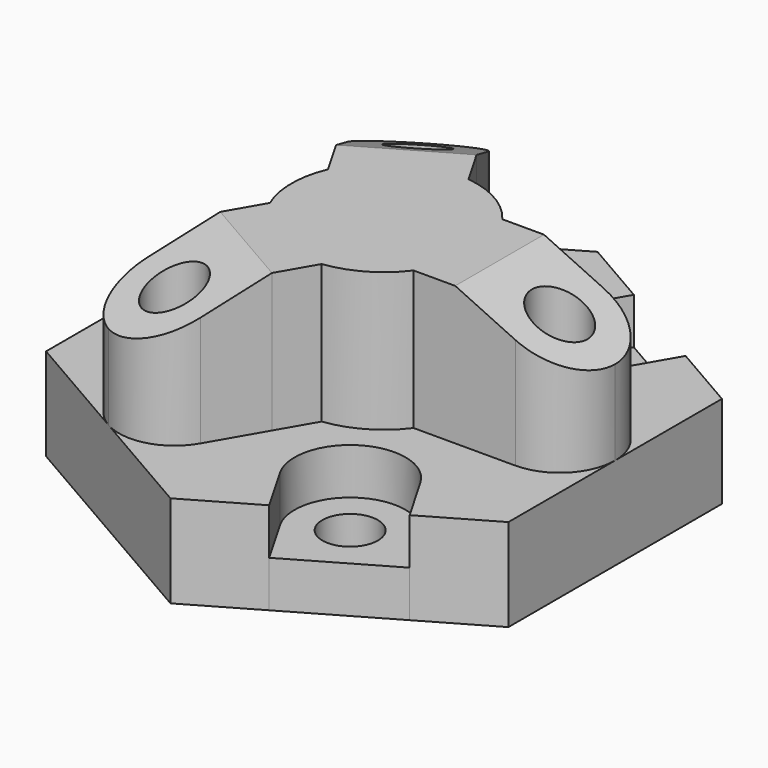
from build123d import *

# Parameters (mm, degrees)
F1_R            = 6
F2_DEPTH        = 20
F3_DEPTH        = 30
F3_DEPTH_BACK   = 20
F4_DEPTH        = 10
F6_DEPTH        = 12.5
F6_COPIES_COUNT = 3


# Not quite as in the source:
# - a pattern or mirror of a feature is missing from the dataset's text; its kind, count and spacing are read off the source's solid


with BuildPart() as f2:
    # F1 (on offset) → F2 (new body, through all)
    with BuildSketch(Plane.XY.offset(20)):
        with BuildLine():
            ThreePointArc((-29.3923048454, 26.9089653438), (-30.5911098969, 36.0147939544), (-24.9999998757, 43.301270261))
            Line((-24.9999998757, 43.301270261), (-50, 28.8675134595))
            Line((-50, 28.8675134595), (-50, 12))
            Line((-50, 12), (-38, 12))
            ThreePointArc((-38, 12), (-26, 0), (-38, -12))
            Line((-38, -12), (-50, -12))
            Line((-50, -12), (-50, -28.8675134595))
            Line((-50, -28.8675134595), (-24.9999998757, -43.301270261))
            ThreePointArc((-24.9999998757, -43.301270261), (-30.5911098969, -36.0147939544), (-29.3923048454, -26.9089653438))
            Line((-29.3923048454, -26.9089653438), (-22.8923048454, -15.6506350946))
            Line((-22.8923048454, -15.6506350946), (-18.3923048454, -7.8564064606))
            ThreePointArc((-18.3923048454, -7.8564064606), (-20, 0), (-18.3923048454, 7.8564064606))
            Line((-18.3923048454, 7.8564064606), (-22.8923048454, 15.6506350946))
            Line((-22.8923048454, 15.6506350946), (-29.3923048454, 26.9089653438))
        make_face()
        with BuildLine():
            Line((-38, 12), (-50, 12))
            Line((-50, 12), (-50, -12))
            Line((-50, -12), (-38, -12))
            ThreePointArc((-38, -12), (-26, 0), (-38, 12))
        make_face()
        with Locations((-38, 0)):
            Circle(F1_R, mode=Mode.SUBTRACT)
    extrude(amount=-F2_DEPTH)



with BuildPart() as f2b:
    # F1 (on offset) → F2, piece 2 (new body, through all)
    with BuildSketch(Plane.XY.offset(20)):
        with BuildLine():
            Line((50, -28.8675134595), (50, 0))
            ThreePointArc((50, 0), (46.4852813742, -8.4852813742), (38, -12))
            Line((38, -12), (25, -12))
            Line((25, -12), (16, -12))
            ThreePointArc((16, -12), (10, -17.3205080757), (2.3923048454, -19.8564064606))
            Line((2.3923048454, -19.8564064606), (-2.1076951546, -27.6506350946))
            Line((-2.1076951546, -27.6506350946), (-8.6076951546, -38.9089653438))
            ThreePointArc((-8.6076951546, -38.9089653438), (-15.8941713895, -44.5000752407), (-24.9999998757, -43.301270261))
            Line((-24.9999998757, -43.301270261), (0, -57.735026919))
            Line((0, -57.735026919), (14.6076951546, -49.3012701892))
            Line((14.6076951546, -49.3012701892), (8.6076951546, -38.9089653438))
            ThreePointArc((8.6076951546, -38.9089653438), (13, -22.5166604984), (29.3923048454, -26.9089653438))
            Line((29.3923048454, -26.9089653438), (35.3923048454, -37.3012701892))
            Line((35.3923048454, -37.3012701892), (50, -28.8675134595))
        make_face()
        with BuildLine():
            Line((14.6076951546, -49.3012701892), (35.3923048454, -37.3012701892))
            Line((35.3923048454, -37.3012701892), (29.3923048454, -26.9089653438))
            ThreePointArc((29.3923048454, -26.9089653438), (13, -22.5166604984), (8.6076951546, -38.9089653438))
            Line((8.6076951546, -38.9089653438), (14.6076951546, -49.3012701892))
        make_face()
        with Locations((19, -32.9089653438)):
            Circle(F1_R, mode=Mode.SUBTRACT)
    extrude(amount=-F2_DEPTH)


with BuildPart() as f2c:
    # F1 (on offset) → F2, piece 3 (new body, through all)
    with BuildSketch(Plane.XY.offset(20)):
        with BuildLine():
            Line((50, 0), (50, 28.8675134595))
            Line((50, 28.8675134595), (35.3923048454, 37.3012701892))
            Line((35.3923048454, 37.3012701892), (29.3923048454, 26.9089653438))
            ThreePointArc((29.3923048454, 26.9089653438), (13, 22.5166604984), (8.6076951546, 38.9089653438))
            Line((8.6076951546, 38.9089653438), (14.6076951546, 49.3012701892))
            Line((14.6076951546, 49.3012701892), (0, 57.735026919))
            Line((0, 57.735026919), (-24.9999998757, 43.301270261))
            ThreePointArc((-24.9999998757, 43.301270261), (-15.8941713895, 44.5000752407), (-8.6076951546, 38.9089653438))
            Line((-8.6076951546, 38.9089653438), (-2.1076951546, 27.6506350946))
            Line((-2.1076951546, 27.6506350946), (2.3923048454, 19.8564064606))
            ThreePointArc((2.3923048454, 19.8564064606), (10, 17.3205080757), (16, 12))
            Line((16, 12), (25, 12))
            Line((25, 12), (38, 12))
            ThreePointArc((38, 12), (46.4852813742, 8.4852813742), (50, 0))
        make_face()
        with BuildLine():
            Line((29.3923048454, 26.9089653438), (35.3923048454, 37.3012701892))
            Line((35.3923048454, 37.3012701892), (14.6076951546, 49.3012701892))
            Line((14.6076951546, 49.3012701892), (8.6076951546, 38.9089653438))
            ThreePointArc((8.6076951546, 38.9089653438), (13, 22.5166604984), (29.3923048454, 26.9089653438))
        make_face()
        with Locations((19, 32.9089653438)):
            Circle(F1_R, mode=Mode.SUBTRACT)
    extrude(amount=-F2_DEPTH)


with BuildPart() as f2_1:
    add(f2.part)

    add(f2b.part)  # F3 merges F2b

    add(f2c.part)  # F3 merges F2c
    # F1 (on offset) → F3 (join, two sides)
    with BuildSketch(Plane.XY.offset(20)) as f3_sk:
        with BuildLine():
            ThreePointArc((-8.6076951546, 38.9089653438), (-15.8941713895, 44.5000752407), (-24.9999998757, 43.301270261))
            ThreePointArc((-24.9999998757, 43.301270261), (-30.5911098969, 36.0147939544), (-29.3923048454, 26.9089653438))
            Line((-29.3923048454, 26.9089653438), (-22.8923048454, 15.6506350946))
            Line((-22.8923048454, 15.6506350946), (-2.1076951546, 27.6506350946))
            Line((-2.1076951546, 27.6506350946), (-8.6076951546, 38.9089653438))
        make_face()
        with Locations((-19, 32.9089653438)):
            Circle(F1_R, mode=Mode.SUBTRACT)
        with BuildLine():
            Line((16, -12), (25, -12))
            Line((25, -12), (25, 12))
            Line((25, 12), (16, 12))
            ThreePointArc((16, 12), (10, 17.3205080757), (2.3923048454, 19.8564064606))
            Line((2.3923048454, 19.8564064606), (-2.1076951546, 27.6506350946))
            Line((-2.1076951546, 27.6506350946), (-22.8923048454, 15.6506350946))
            Line((-22.8923048454, 15.6506350946), (-18.3923048454, 7.8564064606))
            ThreePointArc((-18.3923048454, 7.8564064606), (-20, 0), (-18.3923048454, -7.8564064606))
            Line((-18.3923048454, -7.8564064606), (-22.8923048454, -15.6506350946))
            Line((-22.8923048454, -15.6506350946), (-2.1076951546, -27.6506350946))
            Line((-2.1076951546, -27.6506350946), (2.3923048454, -19.8564064606))
            ThreePointArc((2.3923048454, -19.8564064606), (10, -17.3205080757), (16, -12))
        make_face()
        with BuildLine():
            ThreePointArc((38, -12), (46.4852813742, -8.4852813742), (50, 0))
            ThreePointArc((50, 0), (46.4852813742, 8.4852813742), (38, 12))
            Line((38, 12), (25, 12))
            Line((25, 12), (25, -12))
            Line((25, -12), (38, -12))
        make_face()
        with Locations((38, 0)):
            Circle(F1_R, mode=Mode.SUBTRACT)
        with BuildLine():
            ThreePointArc((-29.3923048454, -26.9089653438), (-30.5911098969, -36.0147939544), (-24.9999998757, -43.301270261))
            ThreePointArc((-24.9999998757, -43.301270261), (-15.8941713895, -44.5000752407), (-8.6076951546, -38.9089653438))
            Line((-8.6076951546, -38.9089653438), (-2.1076951546, -27.6506350946))
            Line((-2.1076951546, -27.6506350946), (-22.8923048454, -15.6506350946))
            Line((-22.8923048454, -15.6506350946), (-29.3923048454, -26.9089653438))
        make_face()
        with Locations((-19, -32.9089653438)):
            Circle(F1_R, mode=Mode.SUBTRACT)
    extrude(amount=F3_DEPTH)
    extrude(f3_sk.sketch, amount=-F3_DEPTH_BACK)

    # F1 (on offset) → F4 (cut)
    with BuildSketch(Plane.XY.offset(20)):
        with BuildLine():
            Line((-38, 12), (-50, 12))
            Line((-50, 12), (-50, -12))
            Line((-50, -12), (-38, -12))
            ThreePointArc((-38, -12), (-26, 0), (-38, 12))
        make_face()
        with Locations((-38, 0)):
            Circle(F1_R, mode=Mode.SUBTRACT)
        with BuildLine():
            Line((14.6076951546, -49.3012701892), (35.3923048454, -37.3012701892))
            Line((35.3923048454, -37.3012701892), (29.3923048454, -26.9089653438))
            ThreePointArc((29.3923048454, -26.9089653438), (13, -22.5166604984), (8.6076951546, -38.9089653438))
            Line((8.6076951546, -38.9089653438), (14.6076951546, -49.3012701892))
        make_face()
        with Locations((19, -32.9089653438)):
            Circle(F1_R, mode=Mode.SUBTRACT)
        with BuildLine():
            Line((29.3923048454, 26.9089653438), (35.3923048454, 37.3012701892))
            Line((35.3923048454, 37.3012701892), (14.6076951546, 49.3012701892))
            Line((14.6076951546, 49.3012701892), (8.6076951546, 38.9089653438))
            ThreePointArc((8.6076951546, 38.9089653438), (13, 22.5166604984), (29.3923048454, 26.9089653438))
        make_face()
        with Locations((19, 32.9089653438)):
            Circle(F1_R, mode=Mode.SUBTRACT)
    extrude(amount=-F4_DEPTH, mode=Mode.SUBTRACT)

    # F5 (on Front) → F6 (cut, symmetric)
    with BuildSketch(Plane.XZ):
        Polygon((50, 50), (25, 50), (50, 38.3423085461), align=None)
    f6 = extrude(amount=F6_DEPTH, both=True, mode=Mode.SUBTRACT)

    # F6_copies: F6 ×3 about axis
    f6_copies_axis = Axis((0, 0, 0), (0, 0, 1))
    for i in range(1, F6_COPIES_COUNT):
        add(f6.rotate(f6_copies_axis, i * 360 / F6_COPIES_COUNT), mode=Mode.SUBTRACT)


solid = f2_1.part
